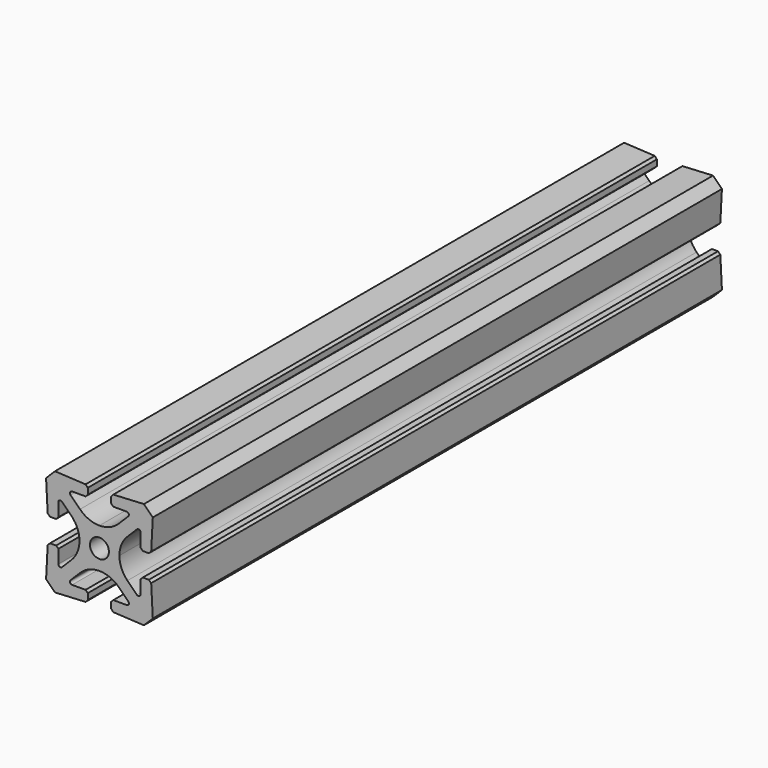
from build123d import *

# Parameters (mm, degrees)
F1_DEPTH = 254


# Not quite as in the source:
# - ends of sketch curves that miss each other by under 0.0002 mm in the source are joined


with BuildPart() as f1:
    # F0 (on Front) → F1 (new body)
    with BuildSketch(Plane.XZ):
        with BuildLine():
            Line((-51.0604008, 40.36949), (-54.2354008, 43.5444646))
            Line((-54.2354008, 43.5444646), (-65.158493, 42.9719994))
            Line((-65.158493, 42.9719994), (-65.9448008, 42.1434006))
            Line((-65.9448008, 42.1434006), (-65.9448008, 39.9630646))
            Line((-65.9448008, 39.9630646), (-65.1573754, 39.17569))
            Line((-65.1573754, 39.17569), (-60.3517716, 39.17569))
            ThreePointArc((-60.3517716, 39.17569), (-59.6477719597, 38.7052864789), (-59.8129689327, 37.8748619331))
            Line((-59.8129689327, 37.8748619331), (-63.1878848, 34.4999818))
            ThreePointArc((-63.1878848, 34.4999818), (-66.3629880966, 32.3740308419), (-70.1104008, 31.6271402404))
            ThreePointArc((-70.1104008, 31.6271402404), (-73.8578286035, 32.3740244671), (-77.0329470659, 34.4999769462))
            Line((-77.0329470659, 34.4999769462), (-80.4078656, 37.8748544))
            ThreePointArc((-80.4078656, 37.8748544), (-80.5730550403, 38.7052864789), (-79.8690554, 39.17569))
            Line((-79.8690554, 39.17569), (-75.0634516, 39.17569))
            Line((-75.0634516, 39.17569), (-74.2760262, 39.9630646))
            Line((-74.2760262, 39.9630646), (-74.2760262, 42.1434006))
            Line((-74.2760262, 42.1434006), (-75.062334, 42.9719994))
            Line((-75.062334, 42.9719994), (-85.9854008, 43.5444646))
            Line((-85.9854008, 43.5444646), (-89.1604008, 40.36949))
            Line((-89.1604008, 40.36949), (-88.5879356, 29.4463978))
            Line((-88.5879356, 29.4463978), (-87.7593368, 28.66009))
            Line((-87.7593368, 28.66009), (-85.5790008, 28.66009))
            Line((-85.5790008, 28.66009), (-84.7916262, 29.4475154))
            Line((-84.7916262, 29.4475154), (-84.7916262, 34.2531192))
            ThreePointArc((-84.7916262, 34.2531192), (-84.3212226789, 34.9571188403), (-83.4907981331, 34.7919218673))
            Line((-83.4907981331, 34.7919218673), (-80.115918, 31.417006))
            ThreePointArc((-80.115918, 31.417006), (-77.9899670419, 28.2419027034), (-77.2430764404, 24.49449))
            ThreePointArc((-77.2430764404, 24.49449), (-77.9899606671, 20.7470621965), (-80.1159131462, 17.5719437341))
            Line((-80.1159131462, 17.5719437341), (-83.4907906, 14.1970252))
            ThreePointArc((-83.4907906, 14.1970252), (-84.3212226789, 14.0318357597), (-84.7916262, 14.7358354))
            Line((-84.7916262, 14.7358354), (-84.7916262, 19.5414392))
            Line((-84.7916262, 19.5414392), (-85.5790008, 20.3288646))
            Line((-85.5790008, 20.3288646), (-87.7593368, 20.3288646))
            Line((-87.7593368, 20.3288646), (-88.5879864, 19.5425314))
            Line((-88.5879864, 19.5425314), (-89.1604262, 8.61949))
            Line((-89.1604262, 8.61949), (-85.9854262, 5.44449))
            Line((-85.9854262, 5.44449), (-75.062334, 6.0169552))
            Line((-75.062334, 6.0169552), (-74.2760262, 6.845554))
            Line((-74.2760262, 6.845554), (-74.2760262, 9.02589))
            Line((-74.2760262, 9.02589), (-75.0634516, 9.8132646))
            Line((-75.0634516, 9.8132646), (-79.8690554, 9.8132646))
            ThreePointArc((-79.8690554, 9.8132646), (-80.5730550403, 10.2836681211), (-80.4078580673, 11.1140926669))
            Line((-80.4078580673, 11.1140926669), (-77.0329422, 14.4889728))
            ThreePointArc((-77.0329422, 14.4889728), (-73.8578286035, 16.6149301329), (-70.1104008, 17.3618143619))
            ThreePointArc((-70.1104008, 17.3618143619), (-66.3629880966, 16.6149237581), (-63.187885217, 14.488972384))
            Line((-63.187885217, 14.488972384), (-59.8129614, 11.1141002))
            ThreePointArc((-59.8129614, 11.1141002), (-59.6477719597, 10.2836681211), (-60.3517716, 9.8132646))
            Line((-60.3517716, 9.8132646), (-65.1573754, 9.8132646))
            Line((-65.1573754, 9.8132646), (-65.9448008, 9.02589))
            Line((-65.9448008, 9.02589), (-65.9448008, 6.845554))
            Line((-65.9448008, 6.845554), (-65.158493, 6.0169552))
            Line((-65.158493, 6.0169552), (-54.2354008, 5.44449))
            Line((-54.2354008, 5.44449), (-51.0604008, 8.61949))
            Line((-51.0604008, 8.61949), (-51.6328406, 19.5425314))
            Line((-51.6328406, 19.5425314), (-52.4614902, 20.3288646))
            Line((-52.4614902, 20.3288646), (-54.6418262, 20.3288646))
            Line((-54.6418262, 20.3288646), (-55.4292008, 19.5414392))
            Line((-55.4292008, 19.5414392), (-55.4292008, 14.7358354))
            ThreePointArc((-55.4292008, 14.7358354), (-55.8996043211, 14.0318357597), (-56.7300288669, 14.1970327327))
            Line((-56.7300288669, 14.1970327327), (-60.104909, 17.5719486))
            ThreePointArc((-60.104909, 17.5719486), (-62.2308663329, 20.7470621965), (-62.9777505619, 24.49449))
            ThreePointArc((-62.9777505619, 24.49449), (-62.2308599581, 28.2419027034), (-60.104908584, 31.417005583))
            Line((-60.104908584, 31.417005583), (-56.7300364, 34.7919294))
            ThreePointArc((-56.7300364, 34.7919294), (-55.8996043211, 34.9571188403), (-55.4292008, 34.2531192))
            Line((-55.4292008, 34.2531192), (-55.4292008, 29.4475154))
            Line((-55.4292008, 29.4475154), (-54.6418262, 28.66009))
            Line((-54.6418262, 28.66009), (-52.4614902, 28.66009))
            Line((-52.4614902, 28.66009), (-51.6328406, 29.4464232))
            Line((-51.6328406, 29.4464232), (-51.0604008, 40.36949))
        make_face()
        with BuildLine():
            ThreePointArc((-73.497059, 24.49449), (-70.1104008, 27.8811482), (-66.7237426, 24.49449))
            ThreePointArc((-66.7237426, 24.49449), (-70.1104008, 21.1078318), (-73.497059, 24.49449))
        make_face(mode=Mode.SUBTRACT)
    extrude(amount=F1_DEPTH)


solid = f1.part
